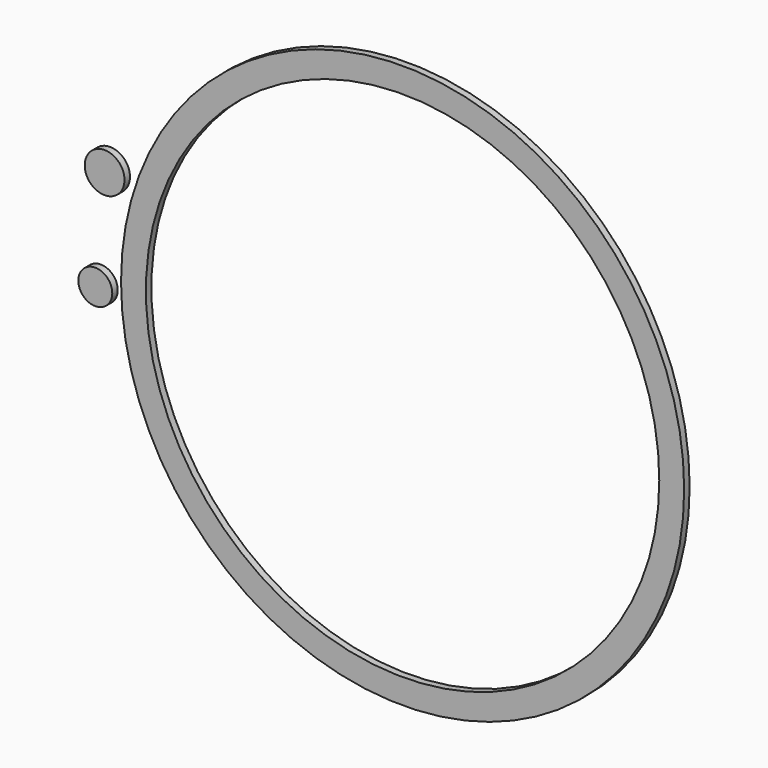
from build123d import *

# Parameters (mm, degrees)
F0_R     = 104.5544645938
F0_R_2   = 95.3072985624
F1_DEPTH = 2.54
F3_R     = 7.3841898205
F4_DEPTH = 2.54
F3_R_2   = 6.30202013
F5_DEPTH = 2.54


# Not quite as in the source:
# - the program builds the solid bodies; features that only make, move or delete a surface that nothing else refers to are left out


with BuildPart() as f1:
    # F0 (on Front) → F1 (new body)
    with BuildSketch(Plane.XZ):
        Circle(F0_R)
        Circle(F0_R_2, mode=Mode.SUBTRACT)
    extrude(amount=F1_DEPTH)


with BuildPart() as f4:
    # F3 (on Front) → F4 (new body)
    with BuildSketch(Plane.XZ):
        with Locations((-110.6478646398, 33.6305089295)):
            Circle(F3_R)
    extrude(amount=F4_DEPTH)


with BuildPart() as f5:
    # F3 (on Front) → F5 (new body)
    with BuildSketch(Plane.XZ):
        with Locations((-114.1076162457, -4.850124009)):
            Circle(F3_R_2)
    extrude(amount=F5_DEPTH)


solid = Compound([f1.part, f4.part, f5.part])
